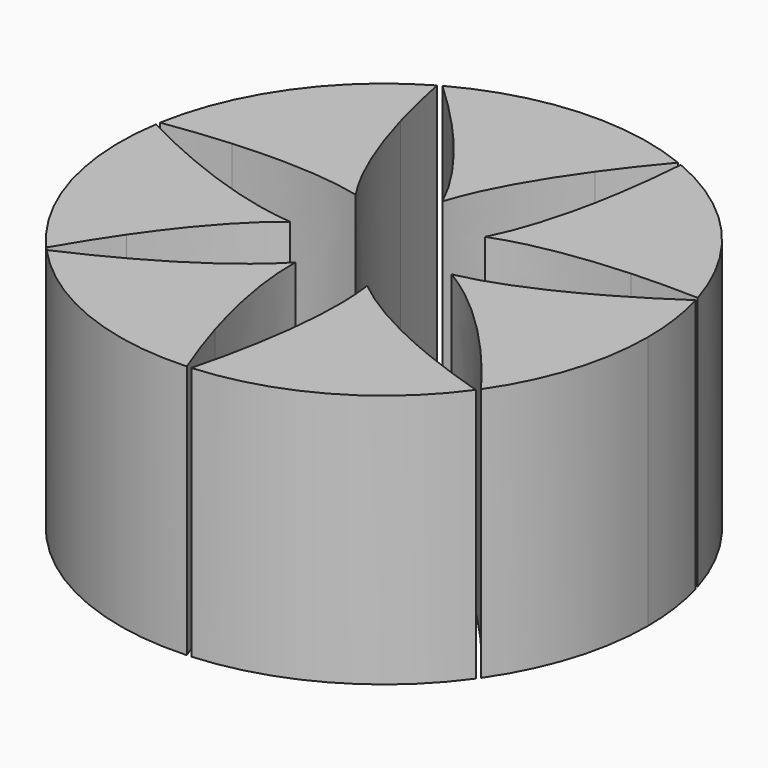
from build123d import *

# Parameters (mm, degrees)
F1_DEPTH = 25


# Not quite as in the source:
# - the program builds the solid bodies; features that only make, move or delete a surface that nothing else refers to are left out


with BuildPart() as f1:
    # F0 (on Top) → F1 (new body)
    with BuildSketch(Plane.XY):
        with BuildLine():
            add(Edge.make_bspline(
                [(-0.4692695513, 7.7720791406), (-2.6156286588, 12.4580584803), (-7.8485191875, 18.1509645982)],
                knots=[0.5135743426, 0.5135743426, 0.5135743426, 0.9861102341, 0.9861102341, 0.9861102341], degree=2, weights=[1, 0.9722183274, 1]))
            add(Edge.make_bspline(
                [(5.6075930615, 18.9634297884), (1.0976837537, 12.682264181), (-0.4692695513, 7.7720791406)],
                knots=[5.2970750731, 5.2970750731, 5.2970750731, 5.7696109645, 5.7696109645, 5.7696109645], degree=2, weights=[1, 0.9722183274, 1]))
            ThreePointArc((5.6075930615, 18.9634297884), (-1.1918315304, 19.739207352), (-7.8485191875, 18.1509645982))
        make_face()
        with BuildLine():
            add(Edge.make_bspline(
                [(-7.8485191875, 18.1509645982), (-9.963024287, 20.4513526823), (-12.4679324412, 22.774157764)],
                knots=[0.9861102341, 0.9861102341, 0.9861102341, 1.1800761223, 1.1800761223, 1.1800761223], degree=2, weights=[1, 0.9953008392, 1]))
            ThreePointArc((-7.8485191875, 18.1509645982), (-1.1918315304, 19.739207352), (5.6075930615, 18.9634297884))
            add(Edge.make_bspline(
                [(9.6371888027, 24.1088405611), (7.4299560897, 21.5015216202), (5.6075930615, 18.9634297884)],
                knots=[5.1031091849, 5.1031091849, 5.1031091849, 5.2970750731, 5.2970750731, 5.2970750731], degree=2, weights=[1, 0.9953008392, 1]))
            ThreePointArc((9.6371888027, 24.1088405611), (-1.5648073137, 25.9164615503), (-12.4679324412, 22.774157764))
        make_face()
    extrude(amount=F1_DEPTH)


with BuildPart() as f1b:
    # F0 (on Top) → F1, piece 2 (new body)
    with BuildSketch(Plane.XY):
        with BuildLine():
            add(Edge.make_bspline(
                [(5.7838713768, 5.2127017923), (8.1092845361, 9.8124532453), (9.297523887, 17.4531607124)],
                knots=[0.5135743426, 0.5135743426, 0.5135743426, 0.9861102341, 0.9861102341, 0.9861102341], degree=2, weights=[1, 0.9722183274, 1]))
            add(Edge.make_bspline(
                [(18.322483511, 7.4393122849), (10.5997880318, 7.0490586649), (5.7838713768, 5.2127017923)],
                knots=[5.2970750731, 5.2970750731, 5.2970750731, 5.7696109645, 5.7696109645, 5.7696109645], degree=2, weights=[1, 0.9722183274, 1]))
            ThreePointArc((18.322483511, 7.4393122849), (14.689638942, 13.239005893), (9.297523887, 17.4531607124))
        make_face()
        with BuildLine():
            ThreePointArc((9.297523887, 17.4531607124), (14.689638942, 13.239005893), (18.322483511, 7.4393122849))
            add(Edge.make_bspline(
                [(24.8577394935, 7.496958616), (21.4430683738, 7.5970058703), (18.322483511, 7.4393122849)],
                knots=[5.1031091849, 5.1031091849, 5.1031091849, 5.2970750731, 5.2970750731, 5.2970750731], degree=2, weights=[1, 0.9953008392, 1]))
            ThreePointArc((24.8577394935, 7.496958616), (19.2866641523, 17.3820650987), (10.0319247992, 23.9472772156))
            add(Edge.make_bspline(
                [(9.297523887, 17.4531607124), (9.7776673475, 20.5406158798), (10.0319247992, 23.9472772156)],
                knots=[0.9861102341, 0.9861102341, 0.9861102341, 1.1800761223, 1.1800761223, 1.1800761223], degree=2, weights=[1, 0.9953008392, 1]))
        make_face()
    extrude(amount=F1_DEPTH)


with BuildPart() as f1c:
    # F0 (on Top) → F1, piece 3 (new body)
    with BuildSketch(Plane.XY):
        with BuildLine():
            add(Edge.make_bspline(
                [(-7.472794591, -2.186954293), (-11.563676812, -5.3222281957), (-15.9494222001, -11.6907100198)],
                knots=[0.5135743426, 0.5135743426, 0.5135743426, 0.9861102341, 0.9861102341, 0.9861102341], degree=2, weights=[1, 0.9722183274, 1]))
            add(Edge.make_bspline(
                [(-19.7357838567, 1.2472388883), (-12.6085509538, -1.75190674), (-7.472794591, -2.186954293)],
                knots=[5.2970750731, 5.2970750731, 5.2970750731, 5.7696109645, 5.7696109645, 5.7696109645], degree=2, weights=[1, 0.9722183274, 1]))
            ThreePointArc((-19.7357838567, 1.2472388883), (-18.9790967465, -5.5543366811), (-15.9494222001, -11.6907100198))
        make_face()
        with BuildLine():
            ThreePointArc((-15.9494222001, -11.6907100198), (-18.9790967465, -5.5543366811), (-19.7357838567, 1.2472388883))
            add(Edge.make_bspline(
                [(-25.6488578464, 4.0308426405), (-22.6157543502, 2.4591329057), (-19.7357838567, 1.2472388883)],
                knots=[5.1031091849, 5.1031091849, 5.1031091849, 5.2970750731, 5.2970750731, 5.2970750731], degree=2, weights=[1, 0.9953008392, 1]))
            ThreePointArc((-25.6488578464, 4.0308426405), (-24.9184793655, -7.2925295563), (-19.4287861092, -17.2230621999))
            add(Edge.make_bspline(
                [(-15.9494222001, -11.6907100198), (-17.7216131025, -14.2640845666), (-19.4287861092, -17.2230621999)],
                knots=[0.9861102341, 0.9861102341, 0.9861102341, 1.1800761223, 1.1800761223, 1.1800761223], degree=2, weights=[1, 0.9953008392, 1]))
        make_face()
    extrude(amount=F1_DEPTH)


with BuildPart() as f1d:
    # F0 (on Top) → F1, piece 4 (new body)
    with BuildSketch(Plane.XY):
        with BuildLine():
            add(Edge.make_bspline(
                [(-2.9493815019, -7.2060097721), (-3.048749004, -12.3592015879), (-0.8041369414, -19.758798877)],
                knots=[0.5135743426, 0.5135743426, 0.5135743426, 0.9861102341, 0.9861102341, 0.9861102341], degree=2, weights=[1, 0.9722183274, 1]))
            add(Edge.make_bspline(
                [(-13.2801905954, -14.652416423), (-6.4916070922, -10.9500580702), (-2.9493815019, -7.2060097721)],
                knots=[5.2970750731, 5.2970750731, 5.2970750731, 5.7696109645, 5.7696109645, 5.7696109645], degree=2, weights=[1, 0.9722183274, 1]))
            ThreePointArc((-13.2801905954, -14.652416423), (-7.4907179885, -18.301527622), (-0.8041369414, -19.758798877))
        make_face()
        with BuildLine():
            ThreePointArc((-0.8041369414, -19.758798877), (-7.4907179885, -18.301527622), (-13.2801905954, -14.652416423))
            add(Edge.make_bspline(
                [(-19.1432409738, -17.5398952745), (-16.023319724, -16.1484644626), (-13.2801905954, -14.652416423)],
                knots=[5.1031091849, 5.1031091849, 5.1031091849, 5.2970750731, 5.2970750731, 5.2970750731], degree=2, weights=[1, 0.9953008392, 1]))
            ThreePointArc((-19.1432409738, -17.5398952745), (-9.8348885682, -24.0288694713), (1.3518822508, -25.9284402847))
            add(Edge.make_bspline(
                [(-0.8041369414, -19.758798877), (0.1028653409, -22.7488263038), (1.3518822508, -25.9284402847)],
                knots=[0.9861102341, 0.9861102341, 0.9861102341, 1.1800761223, 1.1800761223, 1.1800761223], degree=2, weights=[1, 0.9953008392, 1]))
        make_face()
    extrude(amount=F1_DEPTH)


with BuildPart() as f1e:
    # F0 (on Top) → F1, piece 5 (new body)
    with BuildSketch(Plane.XY):
        with BuildLine():
            add(Edge.make_bspline(
                [(-6.3690409359, 4.4789223745), (-11.3709201246, 5.7224915816), (-19.0844672331, 5.1807219294)],
                knots=[0.5135743426, 0.5135743426, 0.5135743426, 0.9861102341, 0.9861102341, 0.9861102341], degree=2, weights=[1, 0.9722183274, 1]))
            add(Edge.make_bspline(
                [(-11.3299293373, 16.2076978777), (-9.2309987796, 8.7654660978), (-6.3690409359, 4.4789223745)],
                knots=[5.2970750731, 5.2970750731, 5.2970750731, 5.7696109645, 5.7696109645, 5.7696109645], degree=2, weights=[1, 0.9722183274, 1]))
            ThreePointArc((-11.3299293373, 16.2076978777), (-16.1758285515, 11.3753830685), (-19.0844672331, 5.1807219294))
        make_face()
        with BuildLine():
            add(Edge.make_bspline(
                [(-19.0844672331, 5.1807219294), (-22.2013554247, 4.9618037835), (-25.579182254, 4.4516330079)],
                knots=[0.9861102341, 0.9861102341, 0.9861102341, 1.1800761223, 1.1800761223, 1.1800761223], degree=2, weights=[1, 0.9953008392, 1]))
            ThreePointArc((-19.0844672331, 5.1807219294), (-16.1758285515, 11.3753830685), (-11.3299293373, 16.2076978777))
            add(Edge.make_bspline(
                [(-12.8403616194, 22.5662738329), (-12.1780646734, 19.2149530389), (-11.3299293373, 16.2076978777)],
                knots=[5.1031091849, 5.1031091849, 5.1031091849, 5.2970750731, 5.2970750731, 5.2970750731], degree=2, weights=[1, 0.9953008392, 1]))
            ThreePointArc((-12.8403616194, 22.5662738329), (-21.2379469562, 14.935233855), (-25.579182254, 4.4516330079))
        make_face()
    extrude(amount=F1_DEPTH)


with BuildPart() as f1f:
    # F0 (on Top) → F1, piece 6 (new body)
    with BuildSketch(Plane.XY):
        with BuildLine():
            add(Edge.make_bspline(
                [(3.7949760146, -6.798792917), (7.7619489872, -10.0894441027), (14.9466798355, -12.9481091738)],
                knots=[0.5135743426, 0.5135743426, 0.5135743426, 0.9861102341, 0.9861102341, 0.9861102341], degree=2, weights=[1, 0.9722183274, 1]))
            add(Edge.make_bspline(
                [(3.1756570507, -19.518503313), (4.5136493145, -11.902592333), (3.7949760146, -6.798792917)],
                knots=[5.2970750731, 5.2970750731, 5.2970750731, 5.7696109645, 5.7696109645, 5.7696109645], degree=2, weights=[1, 0.9722183274, 1]))
            ThreePointArc((3.1756570507, -19.518503313), (9.6383241977, -17.2672949804), (14.9466798355, -12.9481091738))
        make_face()
        with BuildLine():
            ThreePointArc((14.9466798355, -12.9481091738), (9.6383241977, -17.2672949804), (3.1756570507, -19.518503313))
            add(Edge.make_bspline(
                [(1.7776268031, -25.9027342991), (2.6350014706, -22.595938722), (3.1756570507, -19.518503313)],
                knots=[5.1031091849, 5.1031091849, 5.1031091849, 5.2970750731, 5.2970750731, 5.2970750731], degree=2, weights=[1, 0.9953008392, 1]))
            ThreePointArc((1.7776268031, -25.9027342991), (12.6545739161, -22.6709805748), (21.1145557026, -15.1091739914))
            add(Edge.make_bspline(
                [(14.9466798355, -12.9481091738), (17.8498840845, -14.1032378427), (21.1145557026, -15.1091739914)],
                knots=[0.9861102341, 0.9861102341, 0.9861102341, 1.1800761223, 1.1800761223, 1.1800761223], degree=2, weights=[1, 0.9953008392, 1]))
        make_face()
    extrude(amount=F1_DEPTH)


with BuildPart() as f1g:
    # F0 (on Top) → F1, piece 7 (new body)
    with BuildSketch(Plane.XY):
        with BuildLine():
            add(Edge.make_bspline(
                [(7.6816391887, -1.2719463253), (12.7277410761, -0.222129421), (19.4423418396, 3.6127708305)],
                knots=[0.5135743426, 0.5135743426, 0.5135743426, 0.9861102341, 0.9861102341, 0.9861102341], degree=2, weights=[1, 0.9722183274, 1]))
            add(Edge.make_bspline(
                [(17.2401701661, -9.6867591034), (12.1200357257, -3.8922318004), (7.6816391887, -1.2719463253)],
                knots=[5.2970750731, 5.2970750731, 5.2970750731, 5.7696109645, 5.7696109645, 5.7696109645], degree=2, weights=[1, 0.9722183274, 1]))
            ThreePointArc((17.2401701661, -9.6867591034), (19.1309149369, -5.006482094), (19.7751553542, 0))
            ThreePointArc((19.7751553542, 0), (19.6917761973, 1.8140340342), (19.4423418396, 3.6127708305))
        make_face()
        with BuildLine():
            ThreePointArc((19.7751553542, 0), (19.1309149369, -5.006482094), (17.2401701661, -9.6867591034))
            add(Edge.make_bspline(
                [(21.3599053403, -14.760286077), (19.3091128136, -12.0282102505), (17.2401701661, -9.6867591034)],
                knots=[5.1031091849, 5.1031091849, 5.1031091849, 5.2970750731, 5.2970750731, 5.2970750731], degree=2, weights=[1, 0.9953008392, 1]))
            ThreePointArc((21.3599053403, -14.760286077), (24.7860132424, -7.7307922469), (25.9636592417, 0))
            ThreePointArc((25.9636592417, 0), (25.7159472691, 3.5779403673), (24.9775380519, 7.0876084884))
            add(Edge.make_bspline(
                [(19.4423418396, 3.6127708305), (22.1555760412, 5.1623763676), (24.9775380519, 7.0876084884)],
                knots=[0.9861102341, 0.9861102341, 0.9861102341, 1.1800761223, 1.1800761223, 1.1800761223], degree=2, weights=[1, 0.9953008392, 1]))
            ThreePointArc((19.4423418396, 3.6127708305), (19.6917761973, 1.8140340342), (19.7751553542, 0))
        make_face()
    extrude(amount=F1_DEPTH)


solid = Compound([f1.part, f1b.part, f1c.part, f1d.part, f1e.part, f1f.part, f1g.part])
